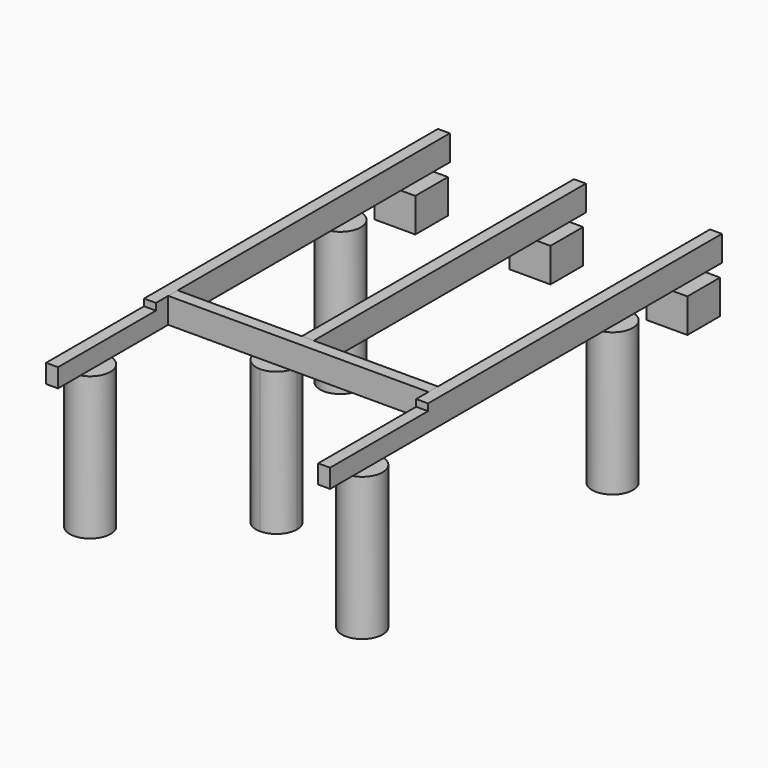
from build123d import *

# Parameters (mm, degrees)
F1_DEPTH  = 190.5
F2_DEPTH  = 190.5
F0_W      = 88.9
F0_H      = 2540
F3_DEPTH  = 190.5
F5_W      = 914.4
F5_H      = 50.8
F6_DEPTH  = 2120.901
F4_W      = 914.4
F4_H      = 50.8
F7_DEPTH  = 2120.901
F8_R      = 152.4
F9_DEPTH  = 1066.8
F10_DEPTH = 1066.8
F11_DEPTH = 1066.8
F12_DEPTH = 1066.8
F13_DEPTH = 1066.8
F14_DEPTH = 190.5
F8_W      = 304.8
F8_H      = 304.8
F15_DEPTH = 254
F8_W_2    = 114.3
F8_W_3    = 88.9
F8_W_4    = 101.6


with BuildPart() as f1:
    # F0 (on Top) → F1 (new body)
    with BuildSketch(Plane.XY):
        Polygon((-1060.45, -1828.8), (-971.55, -1828.8), (-971.55, -800.1), (-971.55, -711.2), (-971.55, 1828.8), (-1060.45, 1828.8), align=None)
    extrude(amount=F1_DEPTH)


with BuildPart() as f2:
    # F0 (on Top) → F2 (new body)
    with BuildSketch(Plane.XY):
        Polygon((971.55, -711.2), (971.55, -800.1), (971.55, -1828.8), (1060.45, -1828.8), (1060.45, 1828.8), (971.55, 1828.8), align=None)
    extrude(amount=F2_DEPTH)


with BuildPart() as f3:
    # F0 (on Top) → F3 (new body)
    with BuildSketch(Plane.XY):
        with Locations((0, 558.8)):
            Rectangle(F0_W, F0_H)
    extrude(amount=F3_DEPTH)


with BuildPart() as f6_tool:
    # F5 (on face) → F6 (new body, through all)
    with BuildSketch(Plane(origin=(-1060.45, 0, 0), x_dir=(0, -1, 0), z_dir=(-1, 0, 0))):
        with Locations((1371.6, 165.1)):
            Rectangle(F5_W, F5_H)
    extrude(amount=-F6_DEPTH)


with BuildPart() as f1_1:
    add(f1.part)

    # F6: cut by f6_tool
    add(f6_tool.part, mode=Mode.SUBTRACT)

    # F4 (on face) → F7 (cut, through all)
    with BuildSketch(Plane.YZ.offset(1060.45)):
        with Locations((-1371.6, 165.1)):
            Rectangle(F4_W, F4_H)
    extrude(amount=-F7_DEPTH, mode=Mode.SUBTRACT)


with BuildPart() as f2_1:
    add(f2.part)

    # F6: cut by f6_tool
    add(f6_tool.part, mode=Mode.SUBTRACT)


with BuildPart() as f9:
    # F8 (on face) → F9 (new body)
    with BuildSketch(Plane(origin=(0, 0, 0), x_dir=(1, 0, 0), z_dir=(0, 0, -1))):
        with Locations((-1016, 1473.2)):
            Circle(F8_R)
    extrude(amount=F9_DEPTH)


with BuildPart() as f10:
    # F8 (on face) → F10 (new body)
    with BuildSketch(Plane(origin=(0, 0, 0), x_dir=(1, 0, 0), z_dir=(0, 0, -1))):
        with Locations((1016, 1473.2)):
            Circle(F8_R)
    extrude(amount=F10_DEPTH)


with BuildPart() as f11:
    # F8 (on face) → F11 (new body)
    with BuildSketch(Plane(origin=(0, 0, 0), x_dir=(1, 0, 0), z_dir=(0, 0, -1))):
        with Locations((1016, -863.6)):
            Circle(F8_R)
    extrude(amount=F11_DEPTH)


with BuildPart() as f12:
    # F8 (on face) → F12 (new body)
    with BuildSketch(Plane(origin=(0, 0, 0), x_dir=(1, 0, 0), z_dir=(0, 0, -1))):
        with Locations((-1016, -863.6)):
            Circle(F8_R)
    extrude(amount=F12_DEPTH)


with BuildPart() as f13:
    # F8 (on face) → F13 (new body)
    with BuildSketch(Plane(origin=(0, 0, 0), x_dir=(1, 0, 0), z_dir=(0, 0, -1))):
        with BuildLine():
            ThreePointArc((-203.2, 596.9), (-95.4369265472, 641.5369265472), (-50.8, 749.3))
            ThreePointArc((-50.8, 749.3), (-95.4369265472, 857.0630734528), (-203.2, 901.7))
            ThreePointArc((-203.2, 901.7), (-310.9630734528, 857.0630734528), (-355.6, 749.3))
            ThreePointArc((-355.6, 749.3), (-310.9630734528, 641.5369265472), (-203.2, 596.9))
        make_face()
    extrude(amount=F13_DEPTH)


with BuildPart() as f14:
    # F0 (on Top) → F14 (new body)
    with BuildSketch(Plane.XY):
        Polygon((-971.55, -711.2), (-971.55, -800.1), (971.55, -800.1), (971.55, -711.2), (44.45, -711.2), (-44.45, -711.2), align=None)
    extrude(amount=F14_DEPTH)


with BuildPart() as f15:
    # F8 (on face) → F15 (new body)
    with BuildSketch(Plane(origin=(0, 0, 0), x_dir=(1, 0, 0), z_dir=(0, 0, -1))):
        with Locations((1016, -1524)):
            Rectangle(F8_W, F8_H)
    extrude(amount=F15_DEPTH)


with BuildPart() as f15b:
    # F8 (on face) → F15, piece 2 (new body)
    with BuildSketch(Plane(origin=(0, 0, 0), x_dir=(1, 0, 0), z_dir=(0, 0, -1))):
        with Locations((-1016, -1524)):
            Rectangle(F8_W, F8_H)
    extrude(amount=F15_DEPTH)


with BuildPart() as f15c:
    # F8 (on face) → F15, piece 3 (new body)
    with BuildSketch(Plane(origin=(0, 0, 0), x_dir=(1, 0, 0), z_dir=(0, 0, -1))):
        with Locations((-101.6, -1524)):
            Rectangle(F8_W_2, F8_H)
        with Locations((0, -1524)):
            Rectangle(F8_W_3, F8_H)
        with Locations((95.25, -1524)):
            Rectangle(F8_W_4, F8_H)
    extrude(amount=F15_DEPTH)


solid = Compound([f3.part, f1_1.part, f2_1.part, f9.part, f10.part, f11.part, f12.part, f13.part, f14.part, f15.part, f15b.part, f15c.part])
